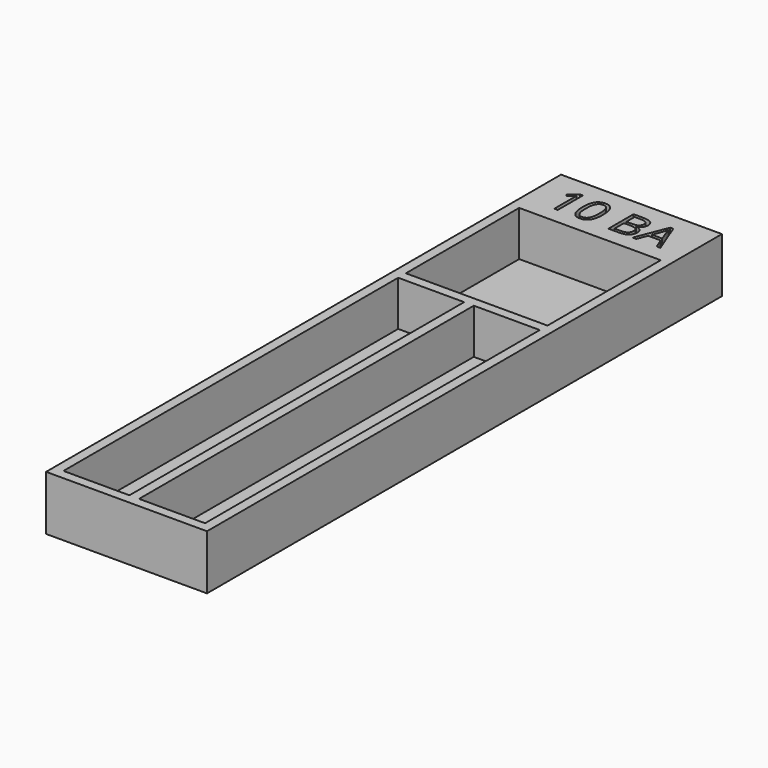
from build123d import *

# Parameters (mm, degrees)
F0_W         = 25
F0_H         = 100
F1_DEPTH     = 0.75
F2_W         = 1.5
F2_H         = 65
F3_DEPTH     = 7
F4_TEXT_SIZE = 6.8289271617
F5_DEPTH     = 1.5


# Not quite as in the source:
# - Text() gives the source's letters only with a copy of the font that has no kerning and outlines rounded to 1/6400 em; it was checked with that copy


with BuildPart() as f1:
    # F0 (on Top) → F1 (new body, symmetric)
    with BuildSketch(Plane.XY):
        with Locations((8.155064851, 32.0954295265)):
            Rectangle(F0_W, F0_H)
    extrude(amount=F1_DEPTH, both=True)

    # F2 (on face) → F3 (join)
    with BuildSketch(Plane.XY.offset(0.75)):
        Polygon((-4.344935149, -17.9045704735), (2.655064851, -17.9045704735), (4.655064851, -17.9045704735), (20.655064851, -17.9045704735), (20.655064851, 82.0954295265), (-4.344935149, 82.0954295265), align=None)
        Polygon((-2.844935149, 50.0954295265), (-2.844935149, 72.0954295265), (19.155064851, 72.0954295265), (19.155064851, 50.0954295265), (19.155064851, 48.5954295265), (19.155064851, -16.4045704735), (8.905064851, -16.4045704735), (7.405064851, -16.4045704735), (-2.844935149, -16.4045704735), (-2.844935149, 48.5954295265), align=None, mode=Mode.SUBTRACT)
        Polygon((19.155064851, 50.0954295265), (-2.844935149, 50.0954295265), (-2.844935149, 48.5954295265), (7.405064851, 48.5954295265), (8.905064851, 48.5954295265), (19.155064851, 48.5954295265), align=None)
        with Locations((8.155064851, 16.0954295265)):
            Rectangle(F2_W, F2_H)
    extrude(amount=F3_DEPTH)

    # F4 (on face) → F5 (cut)
    with BuildSketch(Plane.XY.offset(7.75)):
        with Locations((-1.2309754267, 74.5954295265)):
            Text('10 BA', F4_TEXT_SIZE, font='Open Sans', text_align=(TextAlign.LEFT, TextAlign.BOTTOM))
    extrude(amount=-F5_DEPTH, mode=Mode.SUBTRACT)


solid = f1.part
